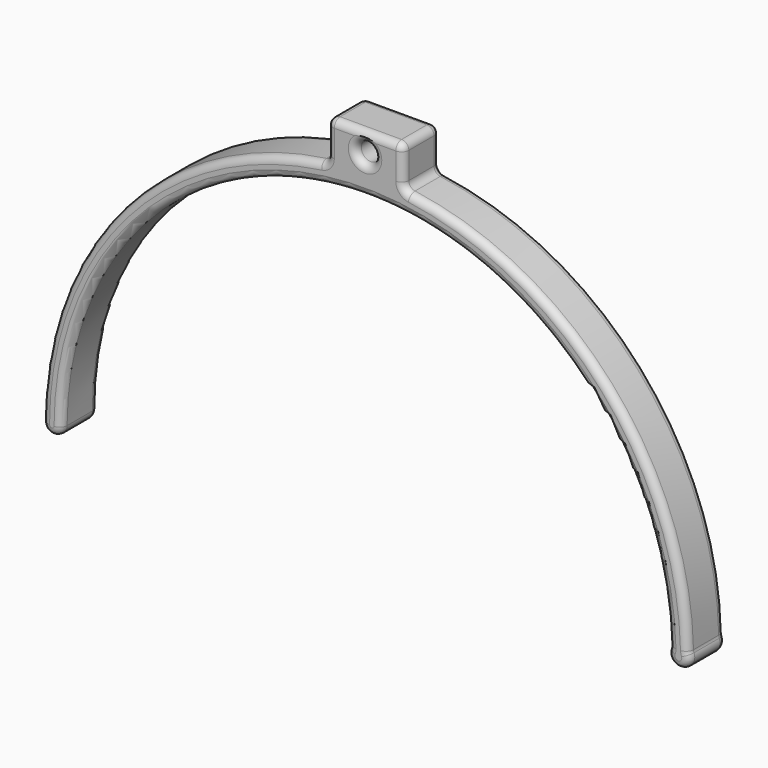
from build123d import *

# Parameters (mm, degrees)
F0_R         = 2.5
F1_DEPTH     = 12.1
F2_T1_DEPTH  = 12.1
F2_T3_DEPTH  = 21.625
F2_T5_DEPTH  = 29.525
F2_T11_DEPTH = 7.0052868996
F2_S15_W     = 1.905
F2_S15_H     = 1.905
F2_T16_DEPTH = 1.905
F2_S21_W     = 1.905
F2_S21_H     = 1.905
F2_T22_DEPTH = 1.905
F2_S27_W     = 1.905
F2_S27_H     = 1.905
F2_T28_DEPTH = 1.905
F2_S33_W     = 1.905
F2_S33_H     = 1.905
F2_T34_DEPTH = 1.905
F2_T38_ANGLE = 82.1263694415
F2_T40_ANGLE = 221.9533464531
F2_T42_ANGLE = 221.9533464531
F2_T44_ANGLE = 80.9830888649
F2_T46_ANGLE = 178.7939525204
F2_T48_ANGLE = 82.1263694415
F2_T50_ANGLE = 180
F2_T52_ANGLE = 180
F2_T54_ANGLE = 80.9830888649
F2_T56_ANGLE = 178.7939525204
F2_T58_ANGLE = 21.5958079127
F2_T60_ANGLE = 20.4203054434
F2_T62_ANGLE = 82.1263694415
F2_T64_ANGLE = 82.1263694415
F2_T66_ANGLE = 82.1263694415
F2_T68_ANGLE = 21.5958079127
F2_T70_ANGLE = 20.4203054434
F2_T72_ANGLE = 82.1263694415


# Not quite as in the source:
# - a fillet or chamfer that OpenCascade refuses, or shapes differently, is made with other operations: its cross-section is extruded or revolved along the edge and cut away or added


with BuildPart() as f1:
    # F0 (on Front) → F1 (new body)
    with BuildSketch(Plane.XZ):
        with BuildLine():
            ThreePointArc((79.9899246621, 1.2696269321), (79.6870956738, 0), (79.9899246621, -1.2696269321))
            ThreePointArc((79.9899246621, -1.2696269321), (80, 0), (79.9899246621, 1.2696269321))
        make_face()
        with BuildLine():
            ThreePointArc((84.9899246621, 1.3087039105), (85, 0), (84.9899246621, -1.3087039105))
            ThreePointArc((84.9899246621, -1.3087039105), (85.3129043262, 0), (84.9899246621, 1.3087039105))
        make_face()
        with BuildLine():
            ThreePointArc((79.9899246621, 1.2696269321), (80, 0), (79.9899246621, -1.2696269321))
            ThreePointArc((79.9899246621, -1.2696269321), (82.478016711, -2.8128184235), (84.9899246621, -1.3087039105))
            ThreePointArc((84.9899246621, -1.3087039105), (85, 0), (84.9899246621, 1.3087039105))
            ThreePointArc((84.9899246621, 1.3087039105), (63.1048014117, 56.9454479199), (10, 84.4097150807))
            Line((10, 84.4097150807), (10, 94.996))
            Line((10, 94.996), (-10, 94.996))
            Line((-10, 94.996), (-10, 84.4097150807))
            ThreePointArc((-10, 84.4097150807), (-61.386574586, 58.7936090115), (-84.7624769577, 6.35))
            ThreePointArc((-84.7624769577, 6.35), (-84.9405984833, 3.177220373), (-85, 0))
            ThreePointArc((-85, 0), (-82.5, -2.5), (-80, 0))
            ThreePointArc((-80, 0), (-0.6348334544, 79.9974811259), (79.9899246621, 1.2696269321))
        make_face()
        with Locations((0, 89.7028575403)):
            Circle(F0_R, mode=Mode.SUBTRACT)
    extrude(amount=F1_DEPTH)

    # F2: fillet of radius 1.905 on 27 edges, made by hand

    # F2_s2 → F2_t1 (join)
    with BuildSketch(Plane.XZ):
        with BuildLine():
            ThreePointArc((11.6440365917, 84.1986722689), (10.4686573715, 84.8343359176), (10, 86.0857131004))
            Line((10, 86.0857131004), (10, 84.4097150807))
            ThreePointArc((10, 84.4097150807), (10.8225327333, 84.3082011742), (11.6440365917, 84.1986722689))
        make_face()
        with BuildLine():
            ThreePointArc((79.8633402498, 0.9800286271), (79.9560670028, 1.3263117777), (79.9822773973, 1.6838356039))
            ThreePointArc((79.9822773973, 1.6838356039), (79.9863691521, 1.4767362182), (79.9899246621, 1.2696269321))
            ThreePointArc((79.9899246621, 1.2696269321), (79.9225618705, 1.1266070465), (79.8633402498, 0.9800286271))
        make_face()
        with BuildLine():
            ThreePointArc((85.1160298765, 1.0338367541), (85.0199774182, 1.3589688139), (84.983078654, 1.6959783275))
            ThreePointArc((84.983078654, 1.6959783275), (84.9867222538, 1.5023450186), (84.9899246621, 1.3087039105))
            ThreePointArc((84.9899246621, 1.3087039105), (85.0566738012, 1.1729662496), (85.1160298765, 1.0338367541))
        make_face()
        with BuildLine():
            ThreePointArc((-10, 86.0857131004), (-10.4686573715, 84.8343359176), (-11.6440365917, 84.1986722689))
            ThreePointArc((-11.6440365917, 84.1986722689), (-10.8225327333, 84.3082011742), (-10, 84.4097150807))
            Line((-10, 84.4097150807), (-10, 86.0857131004))
        make_face()
    extrude(amount=F2_T1_DEPTH)

    # F2_s4 → F2_t3 (cut)
    with BuildSketch(Plane.XZ.offset(-4.7625)):
        with BuildLine():
            ThreePointArc((10, 93.091), (9.4420384182, 94.4380384182), (8.095, 94.996))
            Line((8.095, 94.996), (10, 94.996))
            Line((10, 94.996), (10, 93.091))
        make_face()
        with BuildLine():
            ThreePointArc((-8.095, 94.996), (-9.4420384182, 94.4380384182), (-10, 93.091))
            Line((-10, 93.091), (-10, 94.996))
            Line((-10, 94.996), (-8.095, 94.996))
        make_face()
    extrude(amount=F2_T3_DEPTH, mode=Mode.SUBTRACT)

    # F2_s6 → F2_t5 (cut)
    with BuildSketch(Plane.YZ.offset(-14.7625)):
        with BuildLine():
            ThreePointArc((0, 93.091), (-0.5579615818, 94.4380384182), (-1.905, 94.996))
            Line((-1.905, 94.996), (0, 94.996))
            Line((0, 94.996), (0, 93.091))
        make_face()
        with BuildLine():
            ThreePointArc((-12.1, 93.091), (-11.5420384182, 94.4380384182), (-10.195, 94.996))
            Line((-10.195, 94.996), (-12.1, 94.996))
            Line((-12.1, 94.996), (-12.1, 93.091))
        make_face()
    extrude(amount=F2_T5_DEPTH, mode=Mode.SUBTRACT)

    # F2_s7 → F2_t8 (revolve, cut)
    with BuildSketch(Plane.XY.offset(89.7028575403)):
        with BuildLine():
            ThreePointArc((4.405, -12.1), (3.0579615818, -11.5420384182), (2.5, -10.195))
            Line((2.5, -10.195), (2.5, -12.1))
            Line((2.5, -12.1), (4.405, -12.1))
        make_face()
    revolve(axis=Axis((0, -12.1, 89.7028575403), (0, -1, 0)), mode=Mode.SUBTRACT)

    # F2_s9 → F2_t10 (revolve, cut)
    with BuildSketch(Plane.XY.offset(89.7028575403)):
        with BuildLine():
            ThreePointArc((4.405, 0), (3.0579615818, -0.5579615818), (2.5, -1.905))
            Line((2.5, -1.905), (2.5, 0))
            Line((2.5, 0), (4.405, 0))
        make_face()
    revolve(axis=Axis((0, 0, 89.7028575403), (0, -1, 0)), mode=Mode.SUBTRACT)

    # F2_s12 → F2_t11 (cut)
    with BuildSketch(Plane.XY.offset(86.0857131004)):
        with BuildLine():
            ThreePointArc((8.095, 0), (9.4420384182, -0.5579615818), (10, -1.905))
            Line((10, -1.905), (10, 0))
            Line((10, 0), (8.095, 0))
        make_face()
        with BuildLine():
            ThreePointArc((8.095, -12.1), (9.4420384182, -11.5420384182), (10, -10.195))
            Line((10, -10.195), (10, -12.1))
            Line((10, -12.1), (8.095, -12.1))
        make_face()
        with BuildLine():
            ThreePointArc((-8.095, 0), (-9.4420384182, -0.5579615818), (-10, -1.905))
            Line((-10, -1.905), (-10, 0))
            Line((-10, 0), (-8.095, 0))
        make_face()
        with BuildLine():
            ThreePointArc((-8.095, -12.1), (-9.4420384182, -11.5420384182), (-10, -10.195))
            Line((-10, -10.195), (-10, -12.1))
            Line((-10, -12.1), (-8.095, -12.1))
        make_face()
    extrude(amount=F2_T11_DEPTH, mode=Mode.SUBTRACT)


with BuildPart() as f2_tool14:
    # F2_s15 → F2_t16 (new body)
    with BuildSketch(Plane.XZ.offset(10.195)):
        with Locations((-9.0475, 94.0435)):
            Rectangle(F2_S15_W, F2_S15_H)
    extrude(amount=F2_T16_DEPTH)

    # F2_s17 → F2_t18 (revolve, cut)
    with BuildSketch(Plane(origin=(-8.095, -10.195, 93.091), x_dir=(0.7071067812, 0, -0.7071067812), z_dir=(-0.7071067812, 0, -0.7071067812))):
        with BuildLine():
            ThreePointArc((0, -1.905), (1.905, 0), (0, 1.905))
            Line((0, 1.905), (0, -1.905))
        make_face()
    revolve(axis=Axis((-8.095, -10.195, 93.091), (0, -1, 0)), mode=Mode.SUBTRACT)


with BuildPart() as f1_1:
    add(f1.part)

    # F2_t13: cut F2_tool14
    add(f2_tool14.part, mode=Mode.SUBTRACT)


with BuildPart() as f2_tool20:
    # F2_s21 → F2_t22 (new body)
    with BuildSketch(Plane.XZ.offset(1.905)):
        with Locations((-9.0475, 94.0435)):
            Rectangle(F2_S21_W, F2_S21_H)
    extrude(amount=-F2_T22_DEPTH)

    # F2_s23 → F2_t24 (revolve, cut)
    with BuildSketch(Plane(origin=(-8.095, -1.905, 93.091), x_dir=(0.7071067812, 0, -0.7071067812), z_dir=(0.7071067812, 0, 0.7071067812))):
        with BuildLine():
            ThreePointArc((0, -1.905), (1.905, 0), (0, 1.905))
            Line((0, 1.905), (0, -1.905))
        make_face()
    revolve(axis=Axis((-8.095, -1.905, 93.091), (0, 1, 0)), mode=Mode.SUBTRACT)


with BuildPart() as f1_2:
    add(f1_1.part)

    # F2_t19: cut F2_tool20
    add(f2_tool20.part, mode=Mode.SUBTRACT)


with BuildPart() as f2_tool26:
    # F2_s27 → F2_t28 (new body)
    with BuildSketch(Plane.XZ.offset(10.195)):
        with Locations((9.0475, 94.0435)):
            Rectangle(F2_S27_W, F2_S27_H)
    extrude(amount=F2_T28_DEPTH)

    # F2_s29 → F2_t30 (revolve, cut)
    with BuildSketch(Plane(origin=(8.095, -10.195, 93.091), x_dir=(-0.7071067812, 0, -0.7071067812), z_dir=(-0.7071067812, 0, 0.7071067812))):
        with BuildLine():
            ThreePointArc((0, -1.905), (1.905, 0), (0, 1.905))
            Line((0, 1.905), (0, -1.905))
        make_face()
    revolve(axis=Axis((8.095, -10.195, 93.091), (0, -1, 0)), mode=Mode.SUBTRACT)


with BuildPart() as f1_3:
    add(f1_2.part)

    # F2_t25: cut F2_tool26
    add(f2_tool26.part, mode=Mode.SUBTRACT)


with BuildPart() as f2_tool32:
    # F2_s33 → F2_t34 (new body)
    with BuildSketch(Plane.XZ.offset(1.905)):
        with Locations((9.0475, 94.0435)):
            Rectangle(F2_S33_W, F2_S33_H)
    extrude(amount=-F2_T34_DEPTH)

    # F2_s35 → F2_t36 (revolve, cut)
    with BuildSketch(Plane(origin=(8.095, -1.905, 93.091), x_dir=(-0.7071067812, 0, -0.7071067812), z_dir=(0.7071067812, 0, -0.7071067812))):
        with BuildLine():
            ThreePointArc((0, -1.905), (1.905, 0), (0, 1.905))
            Line((0, 1.905), (0, -1.905))
        make_face()
    revolve(axis=Axis((8.095, -1.905, 93.091), (0, 1, 0)), mode=Mode.SUBTRACT)


with BuildPart() as f1_4:
    add(f1_3.part)

    # F2_t31: cut F2_tool32
    add(f2_tool32.part, mode=Mode.SUBTRACT)

    # F2_s37 → F2_t38 (revolve, cut)
    with BuildSketch(Plane(origin=(0, 0, 0), x_dir=(0, 1, 0), z_dir=(0.9905726149, 0, 0.1369886658))):
        with BuildLine():
            ThreePointArc((-12.1, 83.095), (-11.5420384182, 84.4420384182), (-10.195, 85))
            Line((-10.195, 85), (-12.1, 85))
            Line((-12.1, 85), (-12.1, 83.095))
        make_face()
    revolve(axis=Axis((0, -12.1, 0), (0, -1, 0)), revolution_arc=F2_T38_ANGLE, mode=Mode.SUBTRACT)

    # F2_s39 → F2_t40 (revolve, cut)
    with BuildSketch(Plane(origin=(10.0143219694, 0, 26.9424371201), x_dir=(0, 1, 0), z_dir=(0.3484045362, 0, 0.9373442693))):
        with BuildLine():
            ThreePointArc((-1.905, -74.5179978897), (-0.5579615818, -75.0759594715), (0, -76.4229978897))
            Line((0, -76.4229978897), (0, -74.5179978897))
            Line((0, -74.5179978897), (-1.905, -74.5179978897))
        make_face()
    revolve(axis=Axis((82.5, 0, 0), (0, -1, 0)), revolution_arc=F2_T40_ANGLE, mode=Mode.SUBTRACT)

    # F2_s41 → F2_t42 (revolve, cut)
    with BuildSketch(Plane(origin=(10.0143219694, 0, 26.9424371201), x_dir=(0, 1, 0), z_dir=(0.3484045362, 0, 0.9373442693))):
        with BuildLine():
            ThreePointArc((-10.195, -74.5179978897), (-11.5420384182, -75.0759594715), (-12.1, -76.4229978897))
            Line((-12.1, -76.4229978897), (-12.1, -74.5179978897))
            Line((-12.1, -74.5179978897), (-10.195, -74.5179978897))
        make_face()
    revolve(axis=Axis((82.5, -12.1, 0), (0, -1, 0)), revolution_arc=F2_T42_ANGLE, mode=Mode.SUBTRACT)

    # F2_s43 → F2_t44 (revolve, cut)
    with BuildSketch(Plane(origin=(0, 0, 0), x_dir=(0, 1, 0), z_dir=(0.0199526862, 0, -0.9998009253))):
        with BuildLine():
            ThreePointArc((-12.1, 83.095), (-11.5420384182, 84.4420384182), (-10.195, 85))
            Line((-10.195, 85), (-12.1, 85))
            Line((-12.1, 85), (-12.1, 83.095))
        make_face()
    revolve(axis=Axis((0, -12.1, 0), (0, -1, 0)), revolution_arc=F2_T44_ANGLE, mode=Mode.SUBTRACT)

    # F2_s45 → F2_t46 (revolve, cut)
    with BuildSketch(Plane.XY):
        with BuildLine():
            ThreePointArc((-81.905, -12.1), (-80.5579615818, -11.5420384182), (-80, -10.195))
            Line((-80, -10.195), (-80, -12.1))
            Line((-80, -12.1), (-81.905, -12.1))
        make_face()
    revolve(axis=Axis((0, -12.1, 0), (0, 1, 0)), revolution_arc=F2_T46_ANGLE, mode=Mode.SUBTRACT)

    # F2_s47 → F2_t48 (revolve, cut)
    with BuildSketch(Plane(origin=(0, 0, 0), x_dir=(0, 1, 0), z_dir=(0.9905726149, 0, 0.1369886658))):
        with BuildLine():
            ThreePointArc((0, 83.095), (-0.5579615818, 84.4420384182), (-1.905, 85))
            Line((-1.905, 85), (0, 85))
            Line((0, 85), (0, 83.095))
        make_face()
    revolve(axis=Axis((0, 0, 0), (0, -1, 0)), revolution_arc=F2_T48_ANGLE, mode=Mode.SUBTRACT)

    # F2_s49 → F2_t50 (revolve, cut)
    with BuildSketch(Plane.XY):
        with BuildLine():
            ThreePointArc((-83.095, 0), (-84.4420384182, -0.5579615818), (-85, -1.905))
            Line((-85, -1.905), (-85, 0))
            Line((-85, 0), (-83.095, 0))
        make_face()
    revolve(axis=Axis((-82.5, 0, 0), (0, -1, 0)), revolution_arc=F2_T50_ANGLE, mode=Mode.SUBTRACT)

    # F2_s51 → F2_t52 (revolve, cut)
    with BuildSketch(Plane.XY):
        with BuildLine():
            ThreePointArc((-83.095, -12.1), (-84.4420384182, -11.5420384182), (-85, -10.195))
            Line((-85, -10.195), (-85, -12.1))
            Line((-85, -12.1), (-83.095, -12.1))
        make_face()
    revolve(axis=Axis((-82.5, -12.1, 0), (0, -1, 0)), revolution_arc=F2_T52_ANGLE, mode=Mode.SUBTRACT)

    # F2_s53 → F2_t54 (revolve, cut)
    with BuildSketch(Plane(origin=(0, 0, 0), x_dir=(0, 1, 0), z_dir=(0.0199526862, 0, -0.9998009253))):
        with BuildLine():
            ThreePointArc((0, 83.095), (-0.5579615818, 84.4420384182), (-1.905, 85))
            Line((-1.905, 85), (0, 85))
            Line((0, 85), (0, 83.095))
        make_face()
    revolve(axis=Axis((0, 0, 0), (0, -1, 0)), revolution_arc=F2_T54_ANGLE, mode=Mode.SUBTRACT)

    # F2_s55 → F2_t56 (revolve, cut)
    with BuildSketch(Plane.XY):
        with BuildLine():
            ThreePointArc((-81.905, 0), (-80.5579615818, -0.5579615818), (-80, -1.905))
            Line((-80, -1.905), (-80, 0))
            Line((-80, 0), (-81.905, 0))
        make_face()
    revolve(axis=Axis((0, 0, 0), (0, 1, 0)), revolution_arc=F2_T56_ANGLE, mode=Mode.SUBTRACT)

    # F2_s57 → F2_t58 (revolve, cut)
    with BuildSketch(Plane(origin=(10.0143219694, 0, 26.9424371201), x_dir=(0, 1, 0), z_dir=(-0.3484045362, 0, -0.9373442693))):
        with BuildLine():
            ThreePointArc((0, 76.4229978897), (-0.5579615818, 75.0759594715), (-1.905, 74.5179978897))
            Line((-1.905, 74.5179978897), (0, 74.5179978897))
            Line((0, 74.5179978897), (0, 76.4229978897))
        make_face()
    revolve(axis=Axis((78.0776994168, 0, 1.6437392686), (0, -1, 0)), revolution_arc=F2_T58_ANGLE, mode=Mode.SUBTRACT)

    # F2_s59 → F2_t60 (revolve, cut)
    with BuildSketch(Plane(origin=(11.1441759948, 0, -28.199323768), x_dir=(0, 1, 0), z_dir=(0.3675335647, 0, -0.9300102574))):
        with BuildLine():
            ThreePointArc((0, 77.6337505609), (-0.5579615818, 78.9807889791), (-1.905, 79.5387505609))
            Line((-1.905, 79.5387505609), (0, 79.5387505609))
            Line((0, 79.5387505609), (0, 77.6337505609))
        make_face()
    revolve(axis=Axis((86.8876994168, 0, 1.7339881947), (0, 1, 0)), revolution_arc=F2_T60_ANGLE, mode=Mode.SUBTRACT)

    # F2_s61 → F2_t62 (revolve, cut)
    with BuildSketch(Plane(origin=(0, 0, 0), x_dir=(0, 1, 0), z_dir=(0.9905726149, 0, -0.1369886658))):
        with BuildLine():
            ThreePointArc((0, 83.095), (-0.5579615818, 84.4420384182), (-1.905, 85))
            Line((-1.905, 85), (0, 85))
            Line((0, 85), (0, 83.095))
        make_face()
    revolve(axis=Axis((11.905, 0, 86.0857131004), (0, 1, 0)), revolution_arc=F2_T62_ANGLE, mode=Mode.SUBTRACT)

    # F2_s63 → F2_t64 (revolve, cut)
    with BuildSketch(Plane.XY.offset(86.0857131004)):
        with BuildLine():
            ThreePointArc((-8.095, -12.1), (-9.4420384182, -11.5420384182), (-10, -10.195))
            Line((-10, -10.195), (-10, -12.1))
            Line((-10, -12.1), (-8.095, -12.1))
        make_face()
    revolve(axis=Axis((-11.905, -12.1, 86.0857131004), (0, 1, 0)), revolution_arc=F2_T64_ANGLE, mode=Mode.SUBTRACT)

    # F2_s65 → F2_t66 (revolve, cut)
    with BuildSketch(Plane.XY.offset(86.0857131004)):
        with BuildLine():
            ThreePointArc((-8.095, 0), (-9.4420384182, -0.5579615818), (-10, -1.905))
            Line((-10, -1.905), (-10, 0))
            Line((-10, 0), (-8.095, 0))
        make_face()
    revolve(axis=Axis((-11.905, 0, 86.0857131004), (0, 1, 0)), revolution_arc=F2_T66_ANGLE, mode=Mode.SUBTRACT)

    # F2_s67 → F2_t68 (revolve, cut)
    with BuildSketch(Plane(origin=(10.0143219694, 0, 26.9424371201), x_dir=(0, 1, 0), z_dir=(-0.3484045362, 0, -0.9373442693))):
        with BuildLine():
            ThreePointArc((-12.1, 76.4229978897), (-11.5420384182, 75.0759594715), (-10.195, 74.5179978897))
            Line((-10.195, 74.5179978897), (-12.1, 74.5179978897))
            Line((-12.1, 74.5179978897), (-12.1, 76.4229978897))
        make_face()
    revolve(axis=Axis((78.0776994168, -12.1, 1.6437392686), (0, -1, 0)), revolution_arc=F2_T68_ANGLE, mode=Mode.SUBTRACT)

    # F2_s69 → F2_t70 (revolve, cut)
    with BuildSketch(Plane(origin=(11.1441759948, 0, -28.199323768), x_dir=(0, 1, 0), z_dir=(0.3675335647, 0, -0.9300102574))):
        with BuildLine():
            ThreePointArc((-10.195, 79.5387505609), (-11.5420384182, 78.9807889791), (-12.1, 77.6337505609))
            Line((-12.1, 77.6337505609), (-12.1, 79.5387505609))
            Line((-12.1, 79.5387505609), (-10.195, 79.5387505609))
        make_face()
    revolve(axis=Axis((86.8876994168, -12.1, 1.7339881947), (0, 1, 0)), revolution_arc=F2_T70_ANGLE, mode=Mode.SUBTRACT)

    # F2_s71 → F2_t72 (revolve, cut)
    with BuildSketch(Plane(origin=(0, 0, 0), x_dir=(0, 1, 0), z_dir=(0.9905726149, 0, -0.1369886658))):
        with BuildLine():
            ThreePointArc((-12.1, 83.095), (-11.5420384182, 84.4420384182), (-10.195, 85))
            Line((-10.195, 85), (-12.1, 85))
            Line((-12.1, 85), (-12.1, 83.095))
        make_face()
    revolve(axis=Axis((11.905, -12.1, 86.0857131004), (0, 1, 0)), revolution_arc=F2_T72_ANGLE, mode=Mode.SUBTRACT)


solid = f1_4.part
